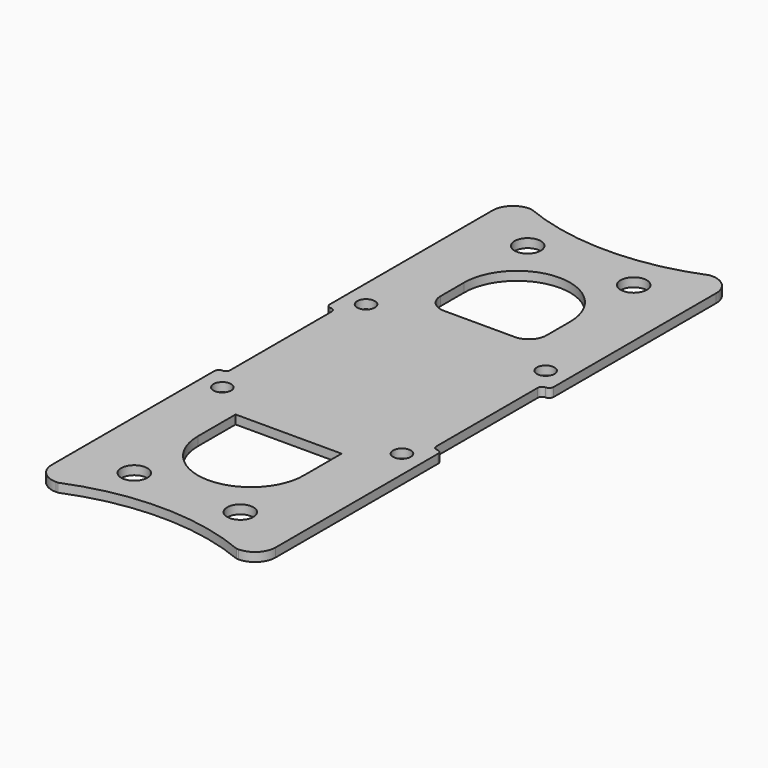
from build123d import *

# Parameters (mm, degrees)
F0_R     = 2.225
F0_R_2   = 1.5
F1_DEPTH = 1.5


# Not quite as in the source:
# - ends of sketch curves that miss each other by under 0.0002 mm in the source are joined


with BuildPart() as f1:
    # F0 (on Top) → F1 (new body)
    with BuildSketch(Plane.XY):
        with BuildLine():
            ThreePointArc((15.5, -50.25), (17.9748737342, -49.2248737342), (19, -46.75))
            Line((19, -46.75), (19, -12.25))
            ThreePointArc((19, -12.25), (18.7803300859, -11.7196699141), (18.25, -11.5))
            ThreePointArc((18.25, -11.5), (17.7196699141, -11.2803300859), (17.5, -10.75))
            Line((17.5, -10.75), (17.5, 10.75))
            ThreePointArc((17.5, 10.75), (17.7196699141, 11.2803300859), (18.25, 11.5))
            ThreePointArc((18.25, 11.5), (18.7803300859, 11.7196699141), (19, 12.25))
            Line((19, 12.25), (19, 46.75))
            ThreePointArc((19, 46.75), (17.9748737342, 49.2248737342), (15.5, 50.25))
            Line((15.5, 50.25), (15.167259, 50.25))
            ThreePointArc((15.167259, 50.25), (0, 47.25), (-15.1672590116, 50.2499999718))
            Line((-15.1672590116, 50.2499999718), (-15.5, 50.25))
            ThreePointArc((-15.5, 50.25), (-17.9748737342, 49.2248737342), (-19, 46.75))
            Line((-19, 46.75), (-19, 12.25))
            ThreePointArc((-19, 12.25), (-18.7803300859, 11.7196699141), (-18.25, 11.5))
            ThreePointArc((-18.25, 11.5), (-17.7196699141, 11.2803300859), (-17.5, 10.75))
            Line((-17.5, 10.75), (-17.5, -10.75))
            ThreePointArc((-17.5, -10.75), (-17.7196699141, -11.2803300859), (-18.25, -11.5))
            ThreePointArc((-18.25, -11.5), (-18.7803300859, -11.7196699141), (-19, -12.25))
            Line((-19, -12.25), (-19, -46.75))
            ThreePointArc((-19, -46.75), (-17.9748737342, -49.2248737342), (-15.5, -50.25))
            Line((-15.5, -50.25), (-15.167259, -50.25))
            ThreePointArc((-15.167259, -50.25), (0, -47.249999), (15.1672593636, -50.2499991168))
            Line((15.1672593636, -50.2499991168), (15.5, -50.25))
        make_face()
        with Locations((-9, -41.75)):
            Circle(F0_R, mode=Mode.SUBTRACT)
        with Locations((-15.25, -15.25)):
            Circle(F0_R_2, mode=Mode.SUBTRACT)
        with Locations((9, -41.75)):
            Circle(F0_R, mode=Mode.SUBTRACT)
        with BuildLine():
            Line((-9, -20.25), (9, -20.25))
            Line((9, -20.25), (9, -28.25))
            ThreePointArc((9, -28.25), (0, -37.25), (-9, -28.25))
            Line((-9, -28.25), (-9, -20.25))
        make_face(mode=Mode.SUBTRACT)
        with Locations((15.25, -15.25)):
            Circle(F0_R_2, mode=Mode.SUBTRACT)
        with Locations((-15.25, 15.25)):
            Circle(F0_R_2, mode=Mode.SUBTRACT)
        with Locations((-9, 41.75)):
            Circle(F0_R, mode=Mode.SUBTRACT)
        with Locations((15.25, 15.25)):
            Circle(F0_R_2, mode=Mode.SUBTRACT)
        with BuildLine():
            ThreePointArc((9, 23.25), (8.1213203436, 21.1286796564), (6, 20.25))
            Line((6, 20.25), (-6, 20.25))
            ThreePointArc((-6, 20.25), (-8.1213203436, 21.1286796564), (-9, 23.25))
            Line((-9, 23.25), (-9, 28.25))
            ThreePointArc((-9, 28.25), (0, 37.25), (9, 28.25))
            Line((9, 28.25), (9, 23.25))
        make_face(mode=Mode.SUBTRACT)
        with Locations((9, 41.75)):
            Circle(F0_R, mode=Mode.SUBTRACT)
    extrude(amount=F1_DEPTH)


solid = f1.part
